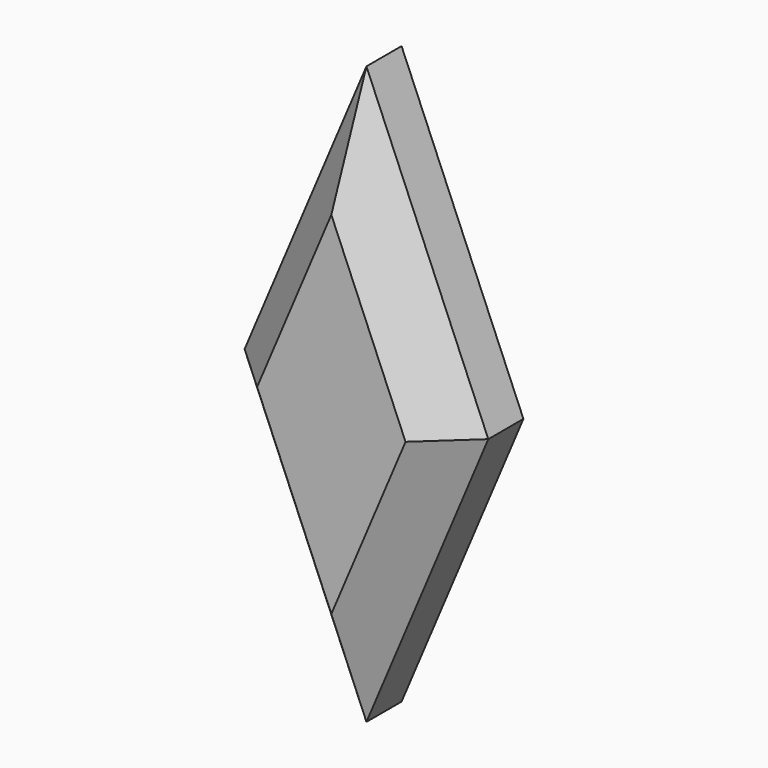
from build123d import *

# Parameters (mm, degrees)
F1_DEPTH = 15
F2_SIZE  = 5


# Not quite as in the source:
# - two fillets or chamfers of one size are made in one step


with BuildPart() as f1:
    # F0 (on Front) → F1 (new body)
    with BuildSketch(Plane.XZ):
        Polygon((13.8800507411, 0), (0, 32.8687280416), (-13.8800498098, 0), (0, -32.8687280416), align=None)
    extrude(amount=F1_DEPTH)

    # F2
    f2_edges = [f1.edges().sort_by_distance(p)[0] for p in [
        (6.940025, -15, 16.434364),
        (-6.940025, -15, 16.434364),
        (-6.940025, -15, -16.434364),
        (6.940025, -15, -16.434364),
        (6.940025, 0, 16.434364),
        (-6.940025, 0, 16.434364),
        (-6.940025, 0, -16.434364),
        (6.940025, 0, -16.434364),
    ]]
    chamfer(f2_edges, length=F2_SIZE)


solid = f1.part
